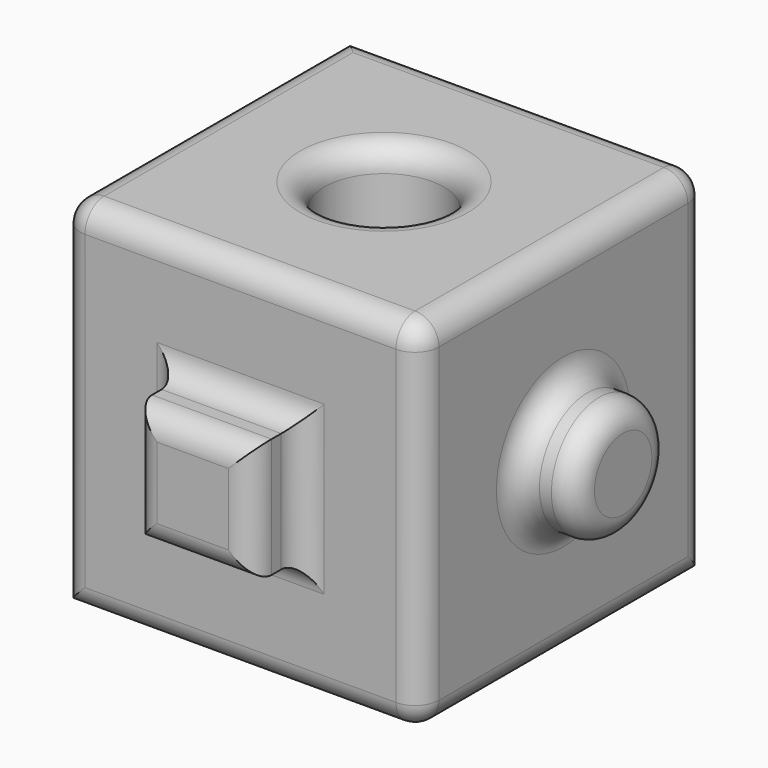
from build123d import *

# Parameters (mm, degrees)
F0_W     = 76.2
F0_H     = 76.2
F1_DEPTH = 76.2
F3_D     = 25.4
F4_W     = 25.4
F4_H     = 25.4
F5_DEPTH = 12.7
F6_R     = 12.7
F7_DEPTH = 12.7
F8_R     = 5.08


with BuildPart() as f1:
    # F0 (on Front) → F1 (new body)
    with BuildSketch(Plane.XZ):
        with Locations((-546.1786431313, 114.5474496245)):
            Rectangle(F0_W, F0_H)
    extrude(amount=F1_DEPTH)

    # F3 (through all)
    with Locations(Plane.XY.offset(152.6474496245)):
        with Locations((-546.1786431313, -38.1)):
            Hole(F3_D / 2)

    # F4 (on face) → F5 (join)
    with BuildSketch(Plane.XZ.offset(76.2)):
        with Locations((-546.1786431313, 114.5474496245)):
            Rectangle(F4_W, F4_H)
    extrude(amount=F5_DEPTH)

    # F6 (on face) → F7 (join)
    with BuildSketch(Plane.YZ.offset(-508.0786431313)):
        with Locations((-38.1, 114.5474496245)):
            Circle(F6_R)
    extrude(amount=F7_DEPTH)

    # F8
    f8_edges = [f1.edges().sort_by_distance(p)[0] for p in [
        (-546.178643, -76.2, 152.64745),
        (-584.278643, -38.1, 152.64745),
        (-546.178643, -88.9, 127.24745),
        (-533.478643, -88.9, 114.54745),
        (-546.178643, -88.9, 101.84745),
        (-558.878643, -88.9, 114.54745),
        (-508.078643, -50.8, 114.54745),
        (-495.378643, -50.8, 114.54745),
        (-584.278643, -76.2, 114.54745),
        (-546.178643, -76.2, 76.44745),
        (-508.078643, -76.2, 114.54745),
        (-533.478643, -76.2, 114.54745),
        (-546.178643, -76.2, 127.24745),
        (-558.878643, -76.2, 114.54745),
        (-546.178643, -76.2, 101.84745),
        (-508.078643, -38.1, 152.64745),
        (-508.078643, 0, 114.54745),
        (-508.078643, -38.1, 76.44745),
        (-546.178643, 0, 152.64745),
        (-558.878643, -38.1, 152.64745),
    ]]
    fillet(f8_edges, radius=F8_R)


solid = f1.part
